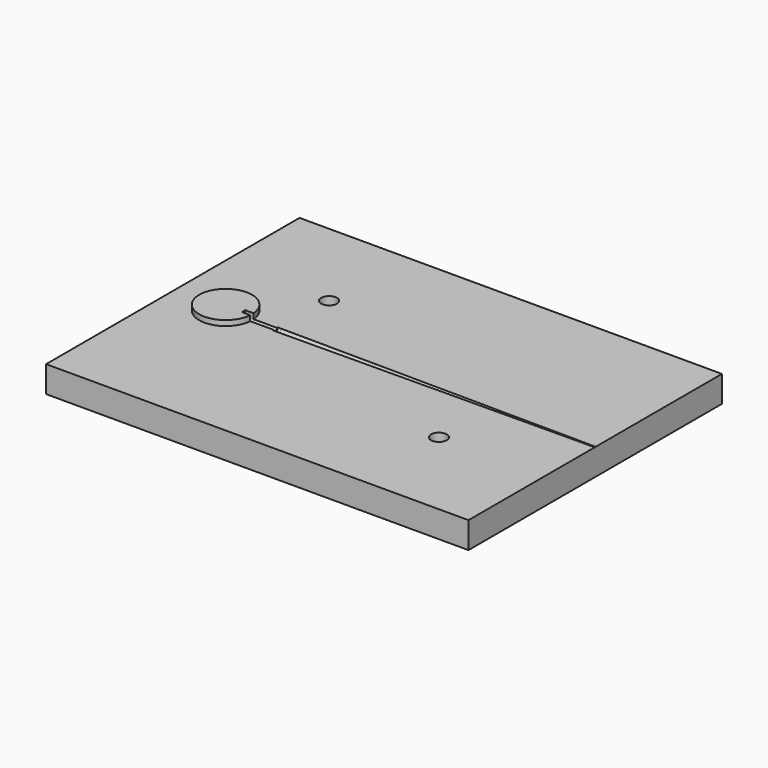
from build123d import *
from build123d import SkipClean  # not in build123d's __all__

# Parameters (mm, degrees)
F0_W          = 400
F0_H          = 300
F1_DEPTH      = 25
F4_R          = 25
F5_DEPTH      = 5
F6_R          = 3
F7_DEPTH      = 3
F9_END_RADIUS = 25
F8_R          = 2
F9_REACH      = 102.6578543495
F10_W         = 11.0047593287
F10_H         = 4
F11_DEPTH     = 5
F14_R         = 7.5
F15_DEPTH     = 25.001


with BuildPart() as f1:
    # F0 (on Top) → F1 (new body)
    with BuildSketch(Plane.XY):
        Rectangle(F0_W, F0_H)
    extrude(amount=F1_DEPTH)

    # F2 (on face) → F3 (revolve, cut)
    with BuildSketch(Plane.XY.offset(25)):
        Polygon((200, 0), (200, 0.5), (-100, 3), (-100, 0), align=None)
    revolve(axis=Axis((50, 0, 25), (1, 0, 0)), mode=Mode.SUBTRACT)

    # F4 (on face) → F5 (join)
    with BuildSketch(Plane.XY.offset(25)):
        with Locations((-150, 0)):
            Circle(F4_R)
    extrude(amount=F5_DEPTH)

    # F6 (on face) → F7 (cut)
    with BuildSketch(Plane.YZ.offset(-100)):
        with Locations((0, 25)):
            Circle(F6_R)
    extrude(amount=-F7_DEPTH, mode=Mode.SUBTRACT)

    f9_end = (Plane(origin=(-150, 0, 27.5), x_dir=(-1, 0, 0), z_dir=(0, 0, -1)) * Cylinder(F9_END_RADIUS, 1207.1140921674, mode=Mode.PRIVATE)).faces().sort_by_distance((-175, 0, 27.5))[0]
    # F8 (on face) → F9 (cut, up to the whole of a round face its end follows)
    with BuildSketch(Plane.YZ.offset(-103)):
        with Locations((0, 25)):
            Circle(F8_R)
    f9_long = extrude(amount=-F9_REACH, mode=Mode.PRIVATE)
    add(split(f9_long, bisect_by=f9_end, keep=Keep.ALL, mode=Mode.PRIVATE).solids().sort_by_distance((-103, 0, 25))[0], mode=Mode.SUBTRACT)

    # F10 (on face) → F11 (cut)
    with BuildSketch(Plane.XY.offset(30)):
        with Locations((-127.4976203357, 0)):
            Rectangle(F10_W, F10_H)
    extrude(amount=-F11_DEPTH, mode=Mode.SUBTRACT)

    # F12 (on face) → F13 (revolve, cut)
    with BuildSketch(Plane.XY.offset(25)):
        with BuildLine():
            Line((-133, 2), (-133, 0))
            Line((-133, 0), (-125, 0))
            ThreePointArc((-125, 0), (-125.020040135, 1.0008022485), (-125.0801284112, 2))
            Line((-125.0801284112, 2), (-133, 2))
        make_face()
        with BuildLine():
            ThreePointArc((-125.0801284112, 2), (-125.020040135, 1.0008022485), (-125, 0))
            Line((-125, 0), (-123.6437782645, 0))
            Line((-123.6437782645, 0), (-123.6437782645, 2))
            Line((-123.6437782645, 2), (-125.0801284112, 2))
        make_face()
    revolve(axis=Axis((-128.3218891323, 0, 25), (1, 0, 0)), mode=Mode.SUBTRACT)

    # F14 (on face) → F15 (cut, through all)
    with BuildSketch(Plane.XY.offset(25)):
        with Locations((100, -60)):
            Circle(F14_R)
        with Locations((-100, 60)):
            Circle(F14_R)
    extrude(amount=-F15_DEPTH, mode=Mode.SUBTRACT)


solid = f1.part
